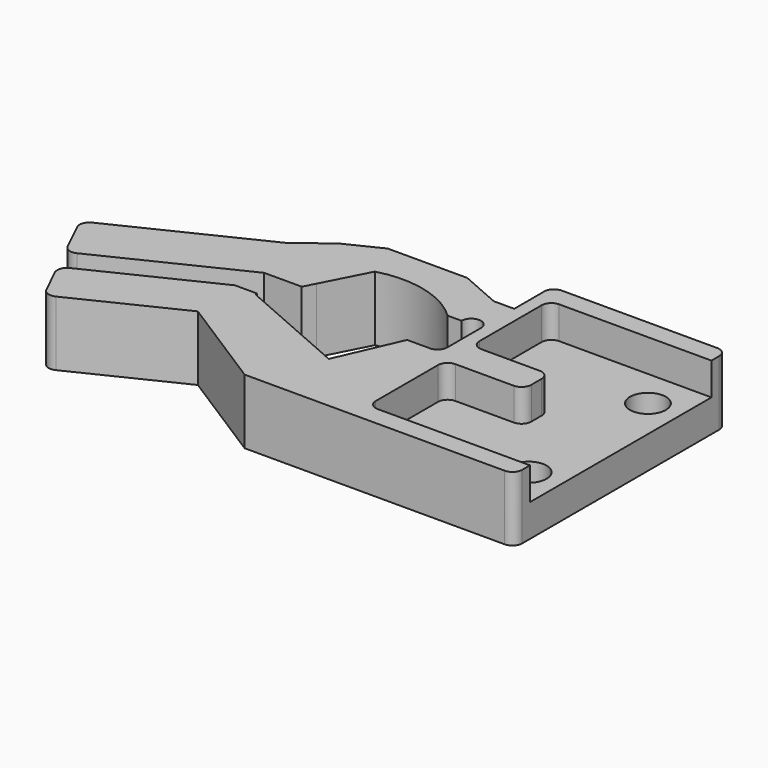
from build123d import *

# Parameters (mm, degrees)
F1_DEPTH = 10
F0_R     = 2.763
F0_R_2   = 2.7634135205
F2_DEPTH = 5


# Not quite as in the source:
# - a feature names something its author has since deleted; it is built from what else it names


with BuildPart() as f1:
    # F0 (on Top) → F1 (new body)
    with BuildSketch(Plane.XY):
        with BuildLine():
            Line((-28.9846330285, 19.3060322961), (-32.4846330285, 19.3060322961))
            Line((-32.4846330285, 19.3060322961), (-36.6950527355, 9.6871775882))
            Line((-36.6950527355, 9.6871775882), (-36.7611596752, 9.5361539153))
            Line((-36.7611596752, 9.5361539153), (-54.1667062895, 17.1550086232))
            Line((-54.1667062895, 17.1550086232), (-54.1667062895, 17.4688580502))
            Line((-54.1667062895, 17.4688580502), (-57.6066188446, 17.4688580502))
            Line((-57.6066188446, 17.4688580502), (-75.9521011029, 8.5636187846))
            ThreePointArc((-75.9521011029, 8.5636187846), (-76.7144296488, 7.7052047395), (-76.6464869407, 6.5591666629))
            Line((-76.6464869407, 6.5591666629), (-75.2652584401, 3.7137290281))
            Line((-75.2652584401, 3.7137290281), (-74.6256538324, 2.3960940233))
            ThreePointArc((-74.6256538324, 2.3960940233), (-73.7672397873, 1.6337654774), (-72.6212017107, 1.7017081855))
            Line((-72.6212017107, 1.7017081855), (-56.8289984312, 9.3675382114))
            Line((-56.8289984312, 9.3675382114), (-42.1148466106, 0))
            Line((-42.1148466106, 0), (-28.5, 0))
            Line((-28.5, 0), (-18.5, 0))
            Line((-18.5, 0), (-1.9846330285, 0))
            ThreePointArc((-1.9846330285, 0), (-0.9239728567, 0.4393398282), (-0.4846330285, 1.5))
            Line((-0.4846330285, 1.5), (-0.4846330285, 3))
            Line((-0.4846330285, 3), (-23.9846330285, 3))
            ThreePointArc((-23.9846330285, 3), (-25.0452932003, 3.4393398282), (-25.4846330285, 4.5))
            Line((-25.4846330285, 4.5), (-25.4846330285, 16.5))
            ThreePointArc((-25.4846330285, 16.5), (-25.0452932003, 17.5606601718), (-23.9846330285, 18))
            Line((-23.9846330285, 18), (-14.9846330285, 18))
            ThreePointArc((-14.9846330285, 18), (-13.9239728567, 18.4393398282), (-13.4846330285, 19.5))
            Line((-13.4846330285, 19.5), (-13.4846330285, 21.5))
            ThreePointArc((-13.4846330285, 21.5), (-13.9239728567, 22.5606601718), (-14.9846330285, 23))
            Line((-14.9846330285, 23), (-23.9846330285, 23))
            ThreePointArc((-23.9846330285, 23), (-25.0452932003, 23.4393398282), (-25.4846330285, 24.5))
            Line((-25.4846330285, 24.5), (-25.4846330285, 36.5))
            ThreePointArc((-25.4846330285, 36.5), (-25.0452932003, 37.5606601718), (-23.9846330285, 38))
            Line((-23.9846330285, 38), (-0.4846330285, 38))
            Line((-0.4846330285, 38), (-0.4846330285, 39.5))
            ThreePointArc((-0.4846330285, 39.5), (-0.9239728567, 40.5606601718), (-1.9846330285, 41))
            Line((-1.9846330285, 41), (-25.4846330285, 41))
            Line((-25.4846330285, 41), (-25.9846330285, 41))
            ThreePointArc((-25.9846330285, 41), (-27.0452932003, 40.5606601718), (-27.4846330285, 39.5))
            Line((-27.4846330285, 39.5), (-27.4846330285, 39.3057436331))
            Line((-27.4846330285, 39.3057436331), (-27.4846330285, 33.7137029542))
            Line((-27.4846330285, 33.7137029542), (-30.6379412534, 33.7137029542))
            Line((-30.6379412534, 33.7137029542), (-36.9315167422, 36.4685625576))
            Line((-36.9315167422, 36.4685625576), (-49.1994071018, 36.4685625576))
            Line((-49.1994071018, 36.4685625576), (-54.7152283086, 33.7718741409))
            Line((-54.7152283086, 33.7718741409), (-59.5651725871, 30.0348878412))
            Line((-59.5651725871, 30.0348878412), (-81.2621656129, 19.502762737))
            ThreePointArc((-81.2621656129, 19.502762737), (-82.0244941588, 18.6443486919), (-81.9565514507, 17.4983106153))
            Line((-81.9565514507, 17.4983106153), (-80.4281407861, 14.3496663292))
            Line((-80.4281407861, 14.3496663292), (-79.683210987, 12.8150532767))
            ThreePointArc((-79.683210987, 12.8150532767), (-78.8247969419, 12.0527247308), (-77.6787588653, 12.1206674389))
            Line((-77.6787588653, 12.1206674389), (-56.8778590157, 22.2178122015))
            Line((-56.8778590157, 22.2178122015), (-51.0782729994, 22.2178122015))
            Line((-51.0782729994, 22.2178122015), (-50.1937510157, 23.9381783364))
            Line((-50.1937510157, 23.9381783364), (-46.6653068671, 30.8008860291))
            ThreePointArc((-46.6653068671, 30.8008860291), (-39.1888505002, 30.8927845811), (-32.6282824459, 27.3060322961))
            Line((-32.6282824459, 27.3060322961), (-30.4846330285, 27.3060322961))
            ThreePointArc((-30.4846330285, 27.3060322961), (-28.9846330285, 28.8060322961), (-27.4846330285, 27.3060322961))
            Line((-27.4846330285, 27.3060322961), (-27.4846330285, 20.8060322961))
            ThreePointArc((-27.4846330285, 20.8060322961), (-27.9239728567, 19.7453721243), (-28.9846330285, 19.3060322961))
        make_face()
    extrude(amount=F1_DEPTH)

    # F0 (on Top) → F2 (join)
    with BuildSketch(Plane.XY):
        with BuildLine():
            Line((-23.9846330285, 3), (-0.4846330285, 3))
            Line((-0.4846330285, 3), (-0.4846330285, 3.0459866499))
            Line((-0.4846330285, 3.0459866499), (-0.4846330285, 37.9540133501))
            Line((-0.4846330285, 37.9540133501), (-0.4846330285, 38))
            Line((-0.4846330285, 38), (-23.9846330285, 38))
            ThreePointArc((-23.9846330285, 38), (-25.0452932003, 37.5606601718), (-25.4846330285, 36.5))
            Line((-25.4846330285, 36.5), (-25.4846330285, 24.5))
            ThreePointArc((-25.4846330285, 24.5), (-25.0452932003, 23.4393398282), (-23.9846330285, 23))
            Line((-23.9846330285, 23), (-14.9846330285, 23))
            ThreePointArc((-14.9846330285, 23), (-13.9239728567, 22.5606601718), (-13.4846330285, 21.5))
            Line((-13.4846330285, 21.5), (-13.4846330285, 19.5))
            ThreePointArc((-13.4846330285, 19.5), (-13.9239728567, 18.4393398282), (-14.9846330285, 18))
            Line((-14.9846330285, 18), (-23.9846330285, 18))
            ThreePointArc((-23.9846330285, 18), (-25.0452932003, 17.5606601718), (-25.4846330285, 16.5))
            Line((-25.4846330285, 16.5), (-25.4846330285, 4.5))
            ThreePointArc((-25.4846330285, 4.5), (-25.0452932003, 3.4393398282), (-23.9846330285, 3))
        make_face()
        with Locations((-5.4846330285, 9)):
            Circle(F0_R, mode=Mode.SUBTRACT)
        with Locations((-5.4846330285, 32)):
            Circle(F0_R_2, mode=Mode.SUBTRACT)
    extrude(amount=F2_DEPTH)


solid = f1.part
